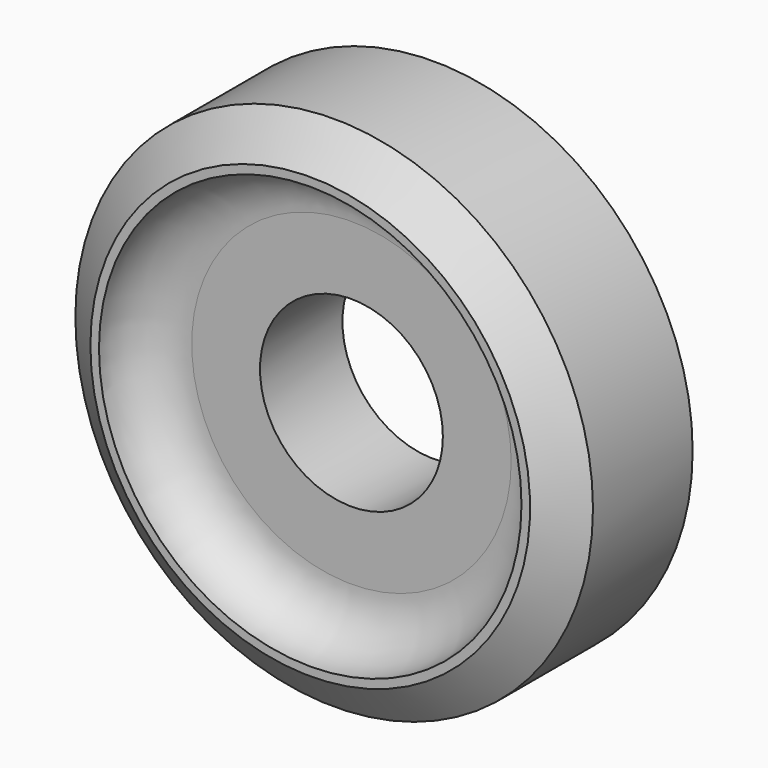
from build123d import *

# Parameters (mm, degrees)
F0_R     = 30.15
F1_DEPTH = 18
F3_R     = 24.61
F4_DEPTH = 6
F5_R     = 5.99999
F6_R     = 10.65
F7_DEPTH = 25


# Not quite as in the source:
# - a fillet or chamfer is up to 0.001 mm smaller than in the source, because OpenCascade refuses the exact size


with BuildPart() as f1:
    # F0 (on Front) → F1 (new body)
    with BuildSketch(Plane.XZ):
        Circle(F0_R)
    extrude(amount=F1_DEPTH)

    # F3 (on face) → F4 (cut)
    with BuildSketch(Plane.XZ.offset(18)):
        Circle(F3_R)
    extrude(amount=-F4_DEPTH, mode=Mode.SUBTRACT)

    # F5 (radius 6 in the source; OpenCascade refuses exactly that, so slightly less here)
    f5_edges = [f1.edges().sort_by_distance(p)[0] for p in [
        (-24.61, -12, 0),
    ]]
    fillet(f5_edges, radius=F5_R)

    # F6 (on face) → F7 (cut)
    with BuildSketch(Plane.XZ.offset(18)):
        Circle(F6_R)
    extrude(amount=-F7_DEPTH, mode=Mode.SUBTRACT)

    # F8 (on Top) → F9 (revolve, cut)
    with BuildSketch(Plane.XY):
        Polygon((-30.15, -18.1521177292), (-25.61, -18), (-30.15, -14.5163354746), align=None)
    revolve(axis=Axis((0, -3.379675094, 0), (0, -1, 0)), mode=Mode.SUBTRACT)


solid = f1.part
